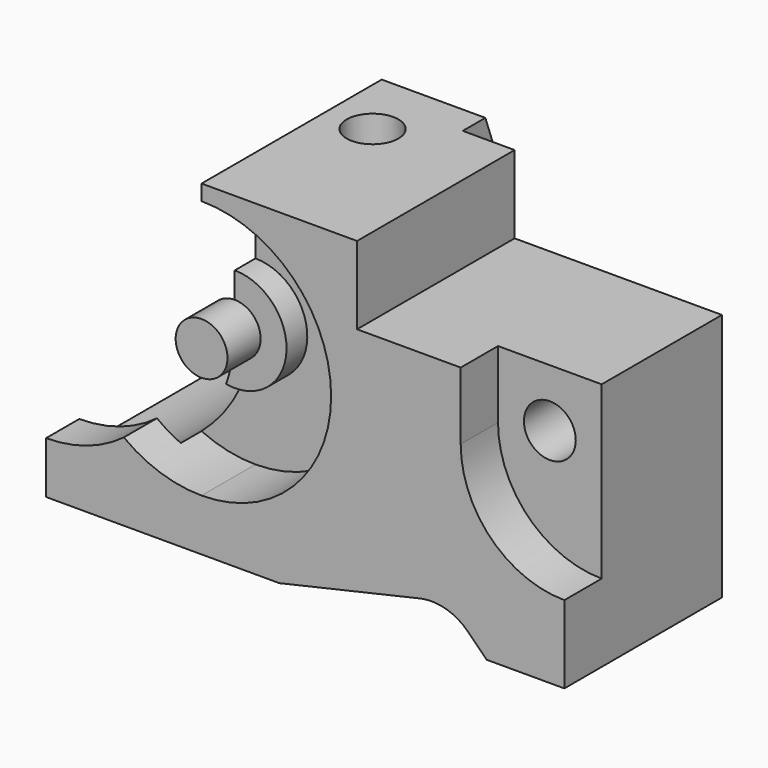
from build123d import *

# Parameters (mm, degrees)
F1_DEPTH  = 50
F3_DEPTH  = 9
F4_R      = 5
F5_DEPTH  = 100
F7_DEPTH  = 8
F9_DEPTH  = 42
F11_DEPTH = 13
F12_W     = 5.5079008639
F12_H     = 3.6583239734
F13_DEPTH = 25
F15_DEPTH = 5
F16_R     = 5
F17_DEPTH = 8
F19_DEPTH = 70.001
F20_W     = 50
F20_H     = 12
F21_DEPTH = 63.001
F22_R     = 5
F23_DEPTH = 63.001
F25_DEPTH = 50.001


with BuildPart() as f1:
    # F0 (on Front) → F1 (new body)
    with BuildSketch(Plane.XZ):
        Polygon((-50, 31.5), (-50, -31.5), (50, -31.5), (50, 16.5), (10, 16.5), (10, 31.5), align=None)
    extrude(amount=F1_DEPTH)

    # F2 (on face) → F3 (cut)
    with BuildSketch(Plane.XZ.offset(50)):
        with BuildLine():
            ThreePointArc((50, -16.5), (64.1421356237, -10.6421356237), (70, 3.5))
            ThreePointArc((70, 3.5), (50, 23.5), (30, 3.5))
            ThreePointArc((30, 3.5), (35.8578643763, -10.6421356237), (50, -16.5))
        make_face()
        with BuildLine():
            Line((30, 16.5), (30, 3.5))
            ThreePointArc((30, 3.5), (31.2386876382, 10.4291527956), (34.8013158464, 16.5))
            Line((34.8013158464, 16.5), (30, 16.5))
        make_face()
    extrude(amount=-F3_DEPTH, mode=Mode.SUBTRACT)

    # F4 (on face) → F5 (cut)
    with BuildSketch(Plane.XZ.offset(41)):
        with Locations((40, 5.378967151)):
            Circle(F4_R)
    extrude(amount=-F5_DEPTH, mode=Mode.SUBTRACT)

    # F6 (on face) → F7 (cut)
    with BuildSketch(Plane.XZ.offset(50)):
        with BuildLine():
            ThreePointArc((-50, -21.5), (-32.3223304703, -14.1776695297), (-25, 3.5))
            ThreePointArc((-25, 3.5), (-67.6776695297, 21.1776695297), (-50, -21.5))
        make_face()
        with BuildLine():
            Line((-50, 31.5), (-50, 28.5))
            ThreePointArc((-50, 28.5), (-32.3223304703, 21.1776695297), (-25, 3.5))
            Line((-25, 3.5), (-25, 31.5))
            Line((-25, 31.5), (-50, 31.5))
        make_face()
    extrude(amount=-F7_DEPTH, mode=Mode.SUBTRACT)

    # F8 (on face) → F9 (cut)
    with BuildSketch(Plane(origin=(0, 0, 0), x_dir=(-1, 0, 0), z_dir=(0, 1, 0))):
        with BuildLine():
            ThreePointArc((50, -26.5), (71.2132034356, -17.7132034356), (80, 3.5))
            ThreePointArc((80, 3.5), (50, 33.5), (20, 3.5))
            ThreePointArc((20, 3.5), (28.7867965644, -17.7132034356), (50, -26.5))
        make_face()
        with BuildLine():
            Line((20, 31.5), (20, 3.5))
            ThreePointArc((20, 3.5), (25.2703630392, 20.4836702684), (39.2296703857, 31.5))
            Line((39.2296703857, 31.5), (20, 31.5))
        make_face()
    extrude(amount=-F9_DEPTH, mode=Mode.SUBTRACT)

    # F10 (on face) → F11 (cut)
    with BuildSketch(Plane.XZ.offset(50)):
        with BuildLine():
            ThreePointArc((-20, -21.5), (-2.3223304703, -14.1776695297), (5, 3.5))
            ThreePointArc((5, 3.5), (-37.6776695297, 21.1776695297), (-20, -21.5))
        make_face()
    extrude(amount=-F11_DEPTH, mode=Mode.SUBTRACT)

    # F12 (on face) → F13 (cut)
    with BuildSketch(Plane(origin=(0, -42, 0), x_dir=(-1, 0, 0), z_dir=(0, 1, 0))):
        with Locations((22.7539504319, 29.6708380133)):
            Rectangle(F12_W, F12_H)
    extrude(amount=-F13_DEPTH, mode=Mode.SUBTRACT)

    # F14 (on face) → F15 (join)
    with BuildSketch(Plane.XZ.offset(37)):
        with BuildLine():
            ThreePointArc((-20, 3.5), (-20.4196010845, -1.5), (-21.6666666667, -6.3601329718))
            ThreePointArc((-21.6666666667, -6.3601329718), (-10.0350281055, 2.6637373972), (-20, 13.5))
            Line((-20, 13.5), (-20, 3.5))
        make_face()
    extrude(amount=F15_DEPTH)

    # F16 (on face) → F17 (join)
    with BuildSketch(Plane.XZ.offset(42)):
        with Locations((-20, 3.5)):
            Circle(F16_R)
    extrude(amount=F17_DEPTH)

    # F18 (on face) → F19 (cut, through all)
    with BuildSketch(Plane(origin=(-20, 0, 0), x_dir=(0, -1, 0), z_dir=(-1, 0, 0))):
        Polygon((0, 31.5), (0, 13.5), (6.5514642168, 31.5), align=None)
    extrude(amount=-F19_DEPTH, mode=Mode.SUBTRACT)

    # F20 (on face) → F21 (cut, through all)
    with BuildSketch(Plane.XY.offset(31.5)):
        with Locations((25, -6)):
            Rectangle(F20_W, F20_H)
    extrude(amount=-F21_DEPTH, mode=Mode.SUBTRACT)

    # F22 (on face) → F23 (cut, through all)
    with BuildSketch(Plane.XY.offset(31.5)):
        with Locations((-11, -20)):
            Circle(F22_R)
    extrude(amount=-F23_DEPTH, mode=Mode.SUBTRACT)

    # F24 (on face) → F25 (cut, through all)
    with BuildSketch(Plane.XZ.offset(50)):
        with BuildLine():
            Line((22.3409673765, -25.2284990706), (-5, -31.5))
            Line((-5, -31.5), (35, -31.5))
            Line((35, -31.5), (31.4479835543, -27.9479835543))
            ThreePointArc((31.4479835543, -27.9479835543), (27.2382101912, -25.437141636), (22.3409673765, -25.2284990706))
        make_face()
    extrude(amount=-F25_DEPTH, mode=Mode.SUBTRACT)


solid = f1.part
